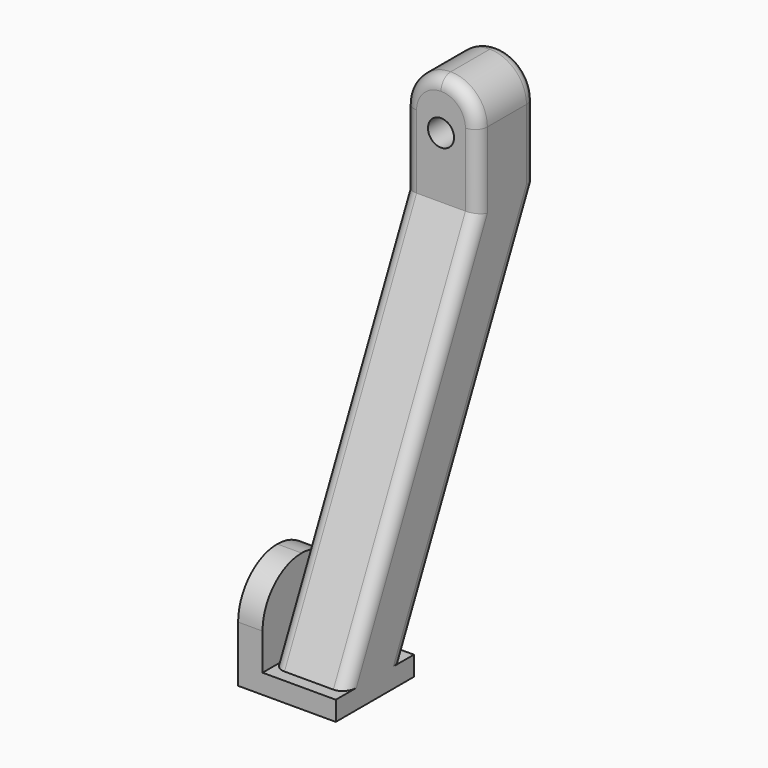
from build123d import *

# Parameters (mm, degrees)
F1_W      = 6
F1_H      = 6
F2_DEPTH  = 1.2
F5_DEPTH  = 2.25
F6_R      = 0.8
F7_DEPTH  = 15.3931915649
F8_R      = 2.24999
F9_R      = 0.75
F11_DEPTH = 1.5


# Not quite as in the source:
# - a fillet or chamfer is up to 0.001 mm smaller than in the source, because OpenCascade refuses the exact size


with BuildPart() as f2:
    # F1 (on Top) → F2 (new body)
    with BuildSketch(Plane.XY):
        with Locations((3, 3)):
            Rectangle(F1_W, F1_H)
    extrude(amount=F2_DEPTH)

    # F4 (on offset) → F5 (join, symmetric)
    with BuildSketch(Plane.YZ.offset(3.75)):
        Polygon((0.75, 1.2), (5.25, 1.2), (15.3921915649, 22.95), (15.3921915649, 29.7), (10.8921915649, 29.7), (10.8921915649, 22.95), align=None)
    extrude(amount=F5_DEPTH, both=True)

    # F6 (on face) → F7 (cut, through all)
    with BuildSketch(Plane(origin=(0, 15.3921915649, 0), x_dir=(-1, 0, 0), z_dir=(0, 1, 0))):
        with Locations((-3.75, 26.7)):
            Circle(F6_R)
    extrude(amount=-F7_DEPTH, mode=Mode.SUBTRACT)

    # F8 (radius 2.25 in the source; OpenCascade refuses exactly that, so slightly less here)
    f8_edges = [f2.edges().sort_by_distance(p)[0] for p in [
        (1.5, 13.142192, 29.7),
        (6, 13.142192, 29.7),
    ]]
    fillet(f8_edges, radius=F8_R)

    # F9
    f9_edges = [f2.edges().sort_by_distance(p)[0] for p in [
        (1.5, 10.321096, 12.075),
        (1.5, 15.392192, 25.200005),
        (5.340993, 15.392192, 29.040993),
        (6, 10.321096, 12.075),
        (1.5, 5.821096, 12.075),
        (1.5, 10.892192, 25.200005),
        (6, 5.821096, 12.075),
    ]]
    fillet(f9_edges, radius=F9_R)

    # F10 (on face) → F11 (join)
    with BuildSketch(Plane(origin=(0, 0, 0), x_dir=(0, -1, 0), z_dir=(-1, 0, 0))):
        with BuildLine():
            Line((-6, 3.45), (-6, 1.2))
            Line((-6, 1.2), (0, 1.2))
            Line((0, 1.2), (0, 3.45))
            ThreePointArc((0, 3.45), (-0.8786796564, 5.5713203436), (-3, 6.45))
            ThreePointArc((-3, 6.45), (-5.1213203436, 5.5713203436), (-6, 3.45))
        make_face()
    extrude(amount=-F11_DEPTH)


solid = f2.part
